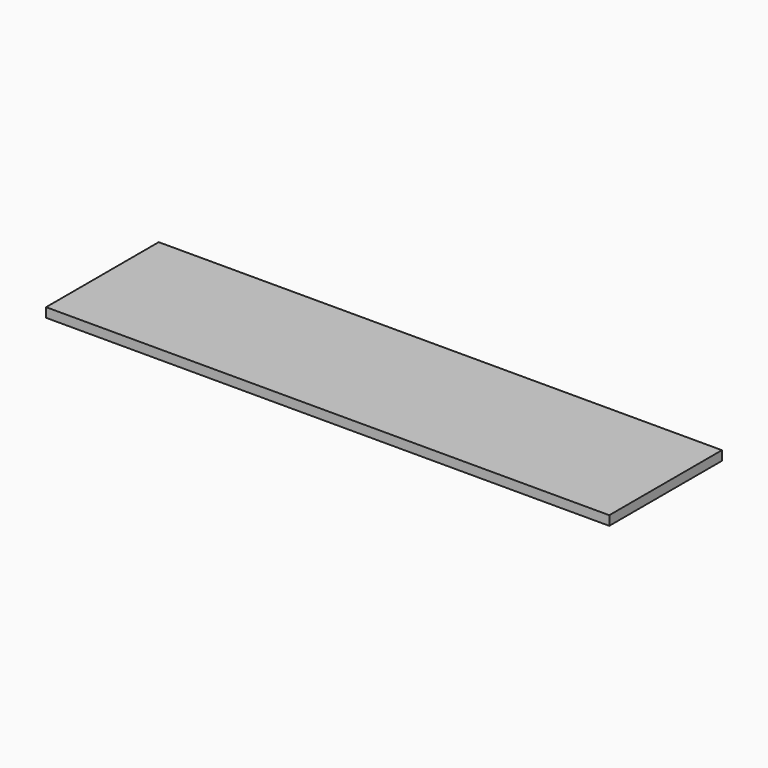
from build123d import *

# Parameters (mm, degrees)
F0_W         = 120
F0_H         = 30
F1_DEPTH     = 2
F2_TEXT_SIZE = 6.4358476715
F3_DEPTH     = 1


# Not quite as in the source:
# - Text() gives the source's letters only with a copy of the font that has no kerning and outlines rounded to 1/6400 em; it was checked with that copy


with BuildPart() as f1:
    # F0 (on Top) → F1 (new body)
    with BuildSketch(Plane.XY):
        with Locations((36.9211384654, -16.2554724235)):
            Rectangle(F0_W, F0_H)
    extrude(amount=F1_DEPTH)

    # F2 (on face) → F3 (cut)
    with BuildSketch(Plane(origin=(0, 0, 0), x_dir=(1, 0, 0), z_dir=(0, 0, -1))):
        with Locations((-13.0788615346, 21.6216621)):
            Text('This is the day that the Lord has made;', F2_TEXT_SIZE, font='Tinos', text_align=(TextAlign.LEFT, TextAlign.BOTTOM))
        with Locations((-0.2071661915, 14.2204372777)):
            Text('let us rejoice and be glad in it.', F2_TEXT_SIZE, font='Tinos', text_align=(TextAlign.LEFT, TextAlign.BOTTOM))
        with Locations((20.7093387409, 6.8192124555)):
            Text('Psalm 118:24', F2_TEXT_SIZE, font='Tinos', text_align=(TextAlign.LEFT, TextAlign.BOTTOM))
    extrude(amount=-F3_DEPTH, mode=Mode.SUBTRACT)


solid = f1.part
